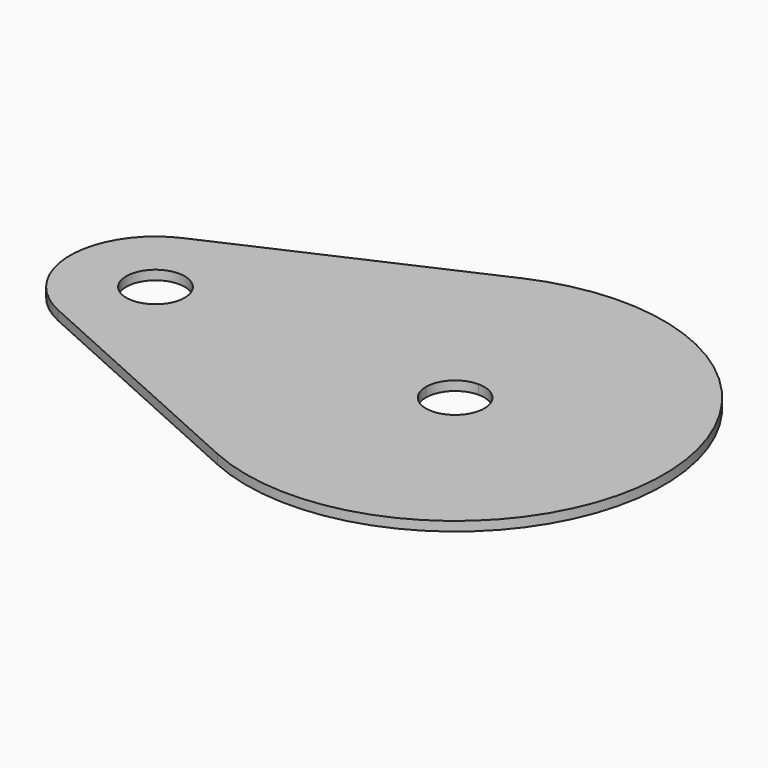
from build123d import *

# Parameters (mm, degrees)
F0_R     = 13.9065
F0_R_2   = 9.906
F1_DEPTH = 3.175


# Not quite as in the source:
# - a length typed as a fraction of an inch, garbled in the dataset ("3 / 203.2 mm" for 3/8 in), is restored


with BuildPart() as f1:
    # F0 (on Top) → F1 (new body)
    with BuildSketch(Plane.XY):
        with BuildLine():
            Line((-29.0468705796, 64.4645603781), (-113.5004093806, 26.4109228888))
            ThreePointArc((-113.5004093806, 26.4109228888), (-130.5681996552, 0), (-113.5004093806, -26.4109228888))
            Line((-113.5004093806, -26.4109228888), (-29.0468705796, -64.4645603781))
            ThreePointArc((-29.0468705796, -64.4645603781), (70.706437014, 0), (-29.0468705796, 64.4645603781))
        make_face()
        with Locations((-101.6, 0)):
            Circle(F0_R, mode=Mode.SUBTRACT)
        with BuildLine():
            ThreePointArc((0, 64.77), (45.7993062175, 45.7993062175), (64.77, 0))
            ThreePointArc((64.77, 0), (45.7993062175, -45.7993062175), (0, -64.77))
            ThreePointArc((0, -64.77), (-45.7993062175, -45.7993062175), (-64.77, 0))
            ThreePointArc((-64.77, 0), (-45.7993062175, 45.7993062175), (0, 64.77))
        make_face(mode=Mode.SUBTRACT)
        with Locations((-101.6, 0)):
            Circle(F0_R)
        with Locations((-101.6, 0)):
            Circle(F0_R_2, mode=Mode.SUBTRACT)
        with BuildLine():
            Line((0, 9.906), (0, 64.77))
            ThreePointArc((0, 64.77), (-45.7993062175, 45.7993062175), (-64.77, 0))
            Line((-64.77, 0), (-9.906, 0))
            ThreePointArc((-9.906, 0), (-7.0045997744, 7.0045997744), (0, 9.906))
        make_face()
        with BuildLine():
            ThreePointArc((-64.77, 0), (-45.7993062175, -45.7993062175), (0, -64.77))
            Line((0, -64.77), (0, -9.906))
            ThreePointArc((0, -9.906), (-7.0045997744, -7.0045997744), (-9.906, 0))
            Line((-9.906, 0), (-64.77, 0))
        make_face()
        with BuildLine():
            ThreePointArc((0, -64.77), (45.7993062175, -45.7993062175), (64.77, 0))
            ThreePointArc((64.77, 0), (45.7993062175, 45.7993062175), (0, 64.77))
            Line((0, 64.77), (0, 9.906))
            ThreePointArc((0, 9.906), (7.0045997744, 7.0045997744), (9.906, 0))
            ThreePointArc((9.906, 0), (7.0045997744, -7.0045997744), (0, -9.906))
            Line((0, -9.906), (0, -64.77))
        make_face()
    extrude(amount=F1_DEPTH)


solid = f1.part
